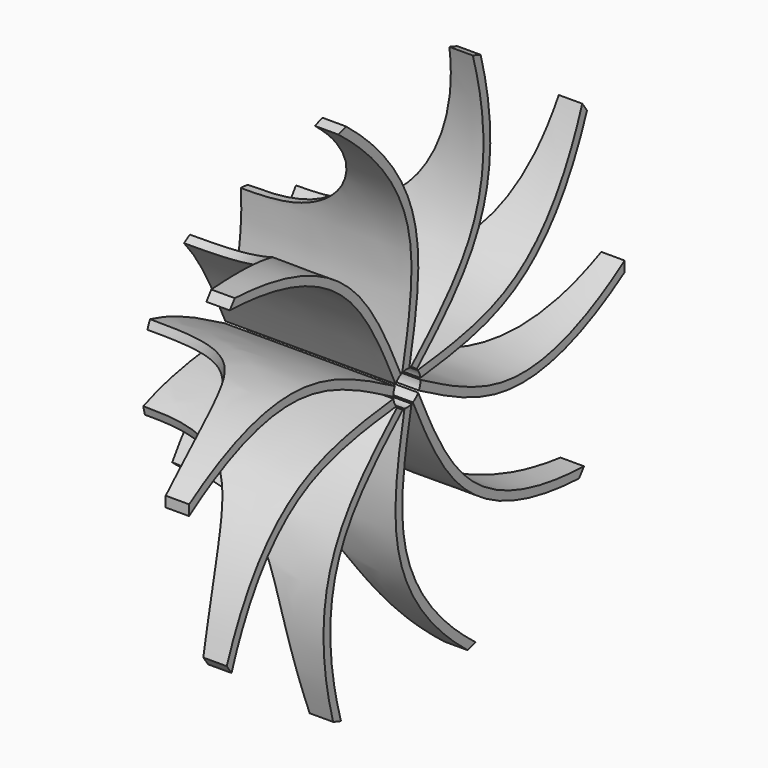
from build123d import *

# Parameters (mm, degrees)
F4_DEPTH = 63.5
F7_W     = 101.6
F7_H     = 95.25
F9_COUNT = 10


# Not quite as in the source:
# - the dataset's text gives a spline's control points without its knots; the knots are read off the source's solid
# - the program builds the solid bodies; features that only make, move or delete a surface that nothing else refers to are left out


with BuildPart() as f4:
    # F3 (on face) → F4 (new body)
    with BuildSketch(Plane.YZ.offset(-69.85)):
        with BuildLine():
            Line((-3.1351240063, 0.501619841), (0, 0))
            add(Edge.make_bspline(
                [(0, 0), (1.524, 9.525), (8.5544527809, 36.1177808283), (3.175, 76.2), (-38.1, 104.775)],
                knots=[0, 0, 0, 0, 0.3810498013, 1, 1, 1, 1], degree=3))
            Line((-38.1, 104.775), (-39.9072416828, 102.1645397915))
            add(Edge.make_bspline(
                [(-3.1351240063, 0.501619841), (-2.6233123042, 3.7004429791), (-1.6763528848, 8.5351817535), (-0.3757040473, 15.2176418807), (0.5436271072, 20.3886593899), (1.2009445195, 24.8649503788), (1.6250143209, 28.5667837946), (1.8828113578, 31.4098189471), (2.0720915767, 34.3210299557), (2.203134959, 38.2740014918), (2.0803406635, 43.3583245115), (1.2889433995, 49.6950440691), (-0.3362482038, 56.2865846902), (-2.9963623183, 63.1583796093), (-8.2095244306, 72.7244631741), (-18.4139273578, 85.4752385435), (-31.7010922987, 96.4833594487), (-39.9072416828, 102.1645397915)],
                knots=[0, 0, 0, 0, 0.125, 0.1875, 0.25, 0.3125, 0.34375, 0.375, 0.40625, 0.4375, 0.5, 0.5625, 0.625, 0.6875, 0.75, 0.875, 1, 1, 1, 1], degree=3))
        make_face()
    extrude(amount=F4_DEPTH)

    # F5 (on Front) → F6 (revolve, cut)
    with BuildSketch(Plane.XZ):
        with BuildLine():
            add(Edge.make_bspline(
                [(-69.85, 44.4434869179), (-69.85, 45.7782377752), (-69.85, 50.2441601154), (-69.85, 58.922774415), (-69.85, 71.7301856825), (-69.85, 85.2766358146), (-69.85, 95.8383724729), (-69.85, 100.9365613061), (-69.85, 102.1645397915)],
                knots=[43.9418670769, 43.9418670769, 43.9418670769, 43.9418670769, 47.9461196486, 57.3396340976, 69.9777099758, 86.368353451, 97.9789844941, 101.6629199505, 101.6629199505, 101.6629199505, 101.6629199505], degree=3))
            add(Edge.make_bspline(
                [(-69.85, 44.4434869179), (-64.0554000113, 44.4362566987), (-48.6920603736, 44.6543312162), (-27.2119468278, 56.6209119816), (-18.1732027709, 83.3044288981), (-15.6718633271, 97.8471549564), (-15.0081717885, 102.1645397915)],
                knots=[0.0363027461, 0.0363027461, 0.0363027461, 0.0363027461, 0.2275299653, 0.4648099055, 0.7405622899, 0.8593134502, 0.8593134502, 0.8593134502, 0.8593134502], degree=3))
            Line((-15.0081717885, 102.1645397915), (-69.85, 102.1645397915))
        make_face()
        with BuildLine():
            add(Edge.make_bspline(
                [(-73.025, 44.45), (-72.0118480085, 44.45), (-70.9500520362, 44.4448595092), (-69.85, 44.4434869179)],
                knots=[0, 0, 0, 0, 0.0363027461, 0.0363027461, 0.0363027461, 0.0363027461], degree=3))
            add(Edge.make_bspline(
                [(-69.85, 44.4434869179), (-69.85, 45.7782377752), (-69.85, 50.2441601154), (-69.85, 58.922774415), (-69.85, 71.7301856825), (-69.85, 85.2766358146), (-69.85, 95.8383724729), (-69.85, 100.9365613061), (-69.85, 102.1645397915)],
                knots=[43.9418670769, 43.9418670769, 43.9418670769, 43.9418670769, 47.9461196486, 57.3396340976, 69.9777099758, 86.368353451, 97.9789844941, 101.6629199505, 101.6629199505, 101.6629199505, 101.6629199505], degree=3))
            Line((-69.85, 102.1645397915), (-15.0081717885, 102.1645397915))
            add(Edge.make_bspline(
                [(-15.0081717885, 102.1645397915), (-14.2218849646, 107.2794201423), (-13.5608613516, 112.3098318902), (-12.7, 117.475)],
                knots=[0.8593134502, 0.8593134502, 0.8593134502, 0.8593134502, 1, 1, 1, 1], degree=3))
            Line((-12.7, 117.475), (-73.025, 117.475))
            Line((-73.025, 117.475), (-73.025, 44.45))
        make_face()
    revolve(axis=Axis((-63.5, 0, 0), (-1, 0, 0)), mode=Mode.SUBTRACT)

    # F7 (on Front) → F8 (revolve, intersect)
    with BuildSketch(Plane.XZ):
        with Locations((-25.4, 53.975)):
            Rectangle(F7_W, F7_H)
    revolve(axis=Axis((-50.8, 0, 0), (-1, 0, 0)), mode=Mode.INTERSECT)


with BuildPart() as f9_1:
    # F9: instance of F4
    add(f4.part.rotate(Axis((-50.8, 0, 0), (-1, 0, 0)), 1 * 360 / F9_COUNT))


with BuildPart() as f9_2:
    # F9: instance of F4
    add(f4.part.rotate(Axis((-50.8, 0, 0), (-1, 0, 0)), 2 * 360 / F9_COUNT))


with BuildPart() as f9_3:
    # F9: instance of F4
    add(f4.part.rotate(Axis((-50.8, 0, 0), (-1, 0, 0)), 3 * 360 / F9_COUNT))


with BuildPart() as f9_4:
    # F9: instance of F4
    add(f4.part.rotate(Axis((-50.8, 0, 0), (-1, 0, 0)), 4 * 360 / F9_COUNT))


with BuildPart() as f9_5:
    # F9: instance of F4
    add(f4.part.rotate(Axis((-50.8, 0, 0), (-1, 0, 0)), 5 * 360 / F9_COUNT))


with BuildPart() as f9_6:
    # F9: instance of F4
    add(f4.part.rotate(Axis((-50.8, 0, 0), (-1, 0, 0)), 6 * 360 / F9_COUNT))


with BuildPart() as f9_7:
    # F9: instance of F4
    add(f4.part.rotate(Axis((-50.8, 0, 0), (-1, 0, 0)), 7 * 360 / F9_COUNT))


with BuildPart() as f9_8:
    # F9: instance of F4
    add(f4.part.rotate(Axis((-50.8, 0, 0), (-1, 0, 0)), 8 * 360 / F9_COUNT))


with BuildPart() as f9_9:
    # F9: instance of F4
    add(f4.part.rotate(Axis((-50.8, 0, 0), (-1, 0, 0)), 9 * 360 / F9_COUNT))


solid = Compound([f4.part, f9_1.part, f9_2.part, f9_3.part, f9_4.part, f9_5.part, f9_6.part, f9_7.part, f9_8.part, f9_9.part])
